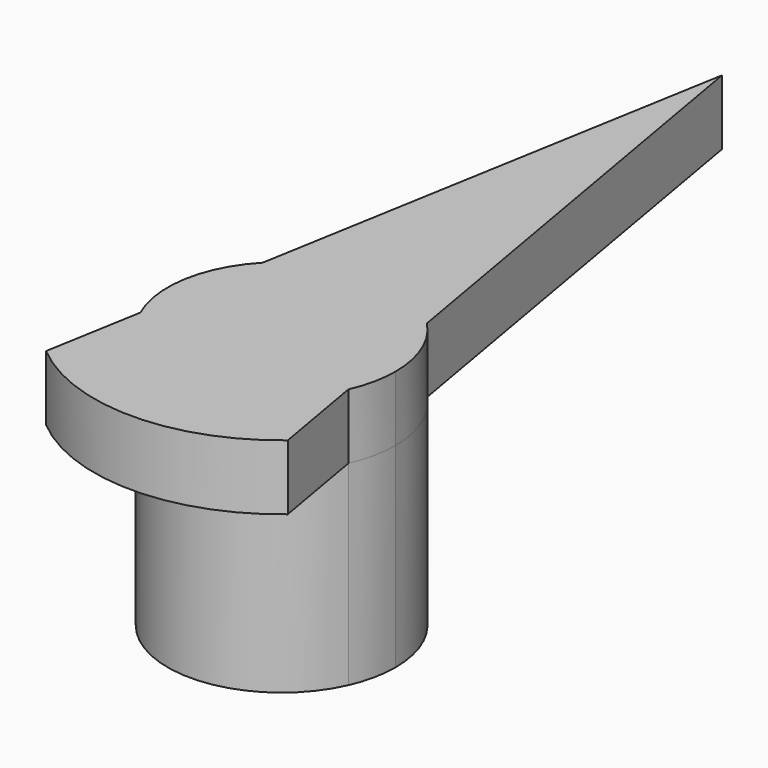
from build123d import *
from build123d import SkipClean  # not in build123d's __all__

# Parameters (mm, degrees)
F1_DEPTH = 2
F2_DEPTH = 6


with BuildPart() as f1:
    # F0 (on Top) → F1 (new body)
    with BuildSketch(Plane.XY):
        with BuildLine():
            Line((-2.522197513, 2.4266272284), (-3.1941037004, -1.430979228))
            ThreePointArc((-3.1941037004, -1.430979228), (0, -3.5), (3.1941037004, -1.430979228))
            Line((3.1941037004, -1.430979228), (2.522197513, 2.4266272284))
            ThreePointArc((2.522197513, 2.4266272284), (0, 3.5), (-2.522197513, 2.4266272284))
        make_face()
        with BuildLine():
            ThreePointArc((2, 1.5), (2.3717082451, 0.790569415), (2.5, 0))
            ThreePointArc((2.5, 0), (2.3717082451, -0.790569415), (2, -1.5))
            ThreePointArc((2, -1.5), (0, -2.5), (-2, -1.5))
            ThreePointArc((-2, -1.5), (-2.5, 0), (-2, 1.5))
            ThreePointArc((-2, 1.5), (0, 2.5), (2, 1.5))
        make_face(mode=Mode.SUBTRACT)
        with BuildLine():
            Line((0, 16.9072877616), (-2.522197513, 2.4266272284))
            ThreePointArc((-2.522197513, 2.4266272284), (0, 3.5), (2.522197513, 2.4266272284))
            Line((2.522197513, 2.4266272284), (0, 16.9072877616))
        make_face()
        with BuildLine():
            Line((-3.1941037004, -1.430979228), (-3.7119607441, -4.4041452929))
            ThreePointArc((-3.7119607441, -4.4041452929), (0, -5.7597871772), (3.7119607441, -4.4041452929))
            Line((3.7119607441, -4.4041452929), (3.1941037004, -1.430979228))
            ThreePointArc((3.1941037004, -1.430979228), (0, -3.5), (-3.1941037004, -1.430979228))
        make_face()
        with BuildLine():
            ThreePointArc((2, -1.5), (2.3717082451, -0.790569415), (2.5, 0))
            ThreePointArc((2.5, 0), (2.3717082451, 0.790569415), (2, 1.5))
            Line((2, 1.5), (-2, 1.5))
            ThreePointArc((-2, 1.5), (-2.5, 0), (-2, -1.5))
            Line((-2, -1.5), (2, -1.5))
        make_face()
        with BuildLine():
            Line((-2, 1.5), (2, 1.5))
            ThreePointArc((2, 1.5), (0, 2.5), (-2, 1.5))
        make_face()
        with BuildLine():
            ThreePointArc((-2, -1.5), (0, -2.5), (2, -1.5))
            Line((2, -1.5), (-2, -1.5))
        make_face()
        with BuildLine():
            Line((2.522197513, 2.4266272284), (3.1941037004, -1.430979228))
            ThreePointArc((3.1941037004, -1.430979228), (3.4226716868, -0.7316546482), (3.5, 0))
            ThreePointArc((3.5, 0), (3.2463588292, 1.3081109862), (2.522197513, 2.4266272284))
        make_face()
        with BuildLine():
            ThreePointArc((-2.522197513, 2.4266272284), (-3.4480874095, 0.6005774025), (-3.1941037004, -1.430979228))
            Line((-3.1941037004, -1.430979228), (-2.522197513, 2.4266272284))
        make_face()
    extrude(amount=F1_DEPTH)

    # F0 (on Top) → F2 (join)
    with BuildSketch(Plane.XY):
        with BuildLine():
            ThreePointArc((-2.522197513, 2.4266272284), (-3.4480874095, 0.6005774025), (-3.1941037004, -1.430979228))
            Line((-3.1941037004, -1.430979228), (-2.522197513, 2.4266272284))
        make_face()
        with BuildLine():
            Line((2.522197513, 2.4266272284), (3.1941037004, -1.430979228))
            ThreePointArc((3.1941037004, -1.430979228), (3.4226716868, -0.7316546482), (3.5, 0))
            ThreePointArc((3.5, 0), (3.2463588292, 1.3081109862), (2.522197513, 2.4266272284))
        make_face()
        with BuildLine():
            Line((-2.522197513, 2.4266272284), (-3.1941037004, -1.430979228))
            ThreePointArc((-3.1941037004, -1.430979228), (0, -3.5), (3.1941037004, -1.430979228))
            Line((3.1941037004, -1.430979228), (2.522197513, 2.4266272284))
            ThreePointArc((2.522197513, 2.4266272284), (0, 3.5), (-2.522197513, 2.4266272284))
        make_face()
        with BuildLine():
            ThreePointArc((2, 1.5), (2.3717082451, 0.790569415), (2.5, 0))
            ThreePointArc((2.5, 0), (2.3717082451, -0.790569415), (2, -1.5))
            ThreePointArc((2, -1.5), (0, -2.5), (-2, -1.5))
            ThreePointArc((-2, -1.5), (-2.5, 0), (-2, 1.5))
            ThreePointArc((-2, 1.5), (0, 2.5), (2, 1.5))
        make_face(mode=Mode.SUBTRACT)
        with BuildLine():
            Line((-2, 1.5), (2, 1.5))
            ThreePointArc((2, 1.5), (0, 2.5), (-2, 1.5))
        make_face()
        with BuildLine():
            ThreePointArc((-2, -1.5), (0, -2.5), (2, -1.5))
            Line((2, -1.5), (-2, -1.5))
        make_face()
    with SkipClean():  # cleaning this boolean's faces spoils the solid; the shape is the same uncleaned
        extrude(amount=-F2_DEPTH)


solid = f1.part
